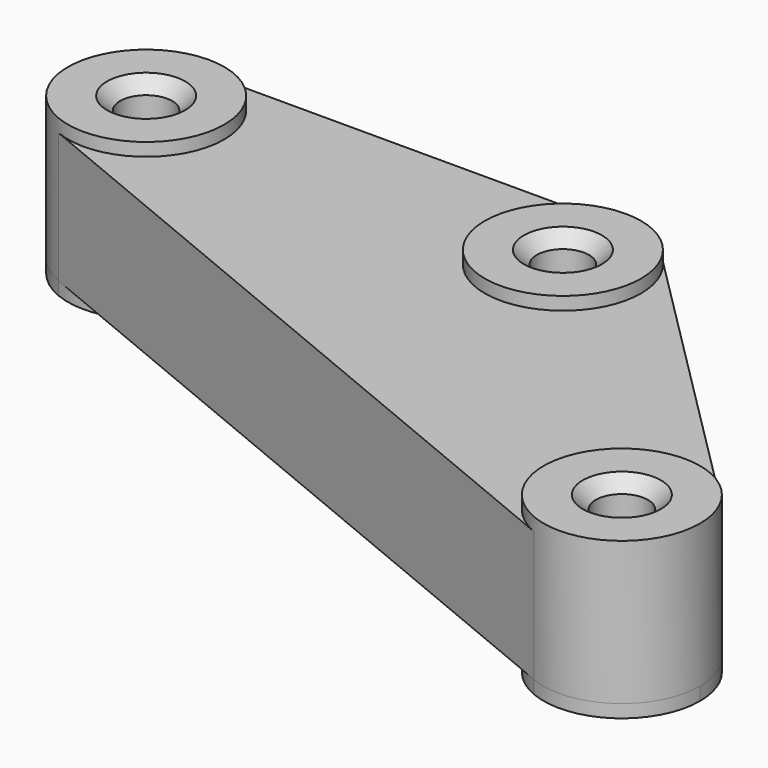
from build123d import *

# Parameters (mm, degrees)
F0_R     = 2
F1_DEPTH = 10
F2_DEPTH = 11
F3_DEPTH = 1


# Not quite as in the source:
# - a fillet or chamfer that OpenCascade refuses, or shapes differently, is made with other operations: its cross-section is extruded or revolved along the edge and cut away or added
# - after a boolean that leaves OpenCascade's solid faulty, fix() repairs it


with BuildPart() as f1:
    # F0 (on Top) → F1 (new body)
    with BuildSketch(Plane.XY):
        with BuildLine():
            Line((26, 0), (6, 0))
            ThreePointArc((6, 0), (3.3334213981, -4.9888176738), (-2.2961005942, -5.5432771951))
            Line((-2.2961005942, -5.5432771951), (52.3313164038, -28.170694193))
            ThreePointArc((52.3313164038, -28.170694193), (48.7427053156, -23.7979589301), (50.3847763109, -18.3847763109))
            Line((50.3847763109, -18.3847763109), (36.2426406871, -4.2426406871))
            ThreePointArc((36.2426406871, -4.2426406871), (29.7038994058, -5.5432771951), (26, 0))
        make_face()
        with BuildLine():
            ThreePointArc((0, 6), (4.2426406871, 4.2426406871), (6, 0))
            Line((6, 0), (26, 0))
            ThreePointArc((26, 0), (27.7573593129, 4.2426406871), (32, 6))
            Line((32, 6), (0, 6))
        make_face()
        with BuildLine():
            ThreePointArc((38, 0), (37.5432771951, -2.2961005942), (36.2426406871, -4.2426406871))
            Line((36.2426406871, -4.2426406871), (50.3847763109, -18.3847763109))
            ThreePointArc((50.3847763109, -18.3847763109), (54.627416998, -16.627416998), (58.8700576851, -18.3847763109))
            Line((58.8700576851, -18.3847763109), (36.2426406871, 4.2426406871))
            ThreePointArc((36.2426406871, 4.2426406871), (37.5432771951, 2.2961005942), (38, 0))
        make_face()
        with BuildLine():
            ThreePointArc((-2.2961005942, -5.5432771951), (3.3334213981, -4.9888176738), (6, 0))
            ThreePointArc((6, 0), (4.2426406871, 4.2426406871), (0, 6))
            ThreePointArc((0, 6), (-5.8847116824, 1.1705419321), (-2.2961005942, -5.5432771951))
        make_face()
        Circle(F0_R, mode=Mode.SUBTRACT)
        with BuildLine():
            Line((30, 0), (26, 0))
            ThreePointArc((26, 0), (29.7038994058, -5.5432771951), (36.2426406871, -4.2426406871))
            Line((36.2426406871, -4.2426406871), (33.4142135624, -1.4142135624))
            ThreePointArc((33.4142135624, -1.4142135624), (31.2346331353, -1.847759065), (30, 0))
        make_face()
        with BuildLine():
            ThreePointArc((32, 6), (27.7573593129, 4.2426406871), (26, 0))
            Line((26, 0), (30, 0))
            ThreePointArc((30, 0), (32, 2), (34, 0))
            ThreePointArc((34, 0), (33.847759065, -0.7653668647), (33.4142135624, -1.4142135624))
            Line((33.4142135624, -1.4142135624), (36.2426406871, -4.2426406871))
            ThreePointArc((36.2426406871, -4.2426406871), (37.5432771951, -2.2961005942), (38, 0))
            ThreePointArc((38, 0), (37.5432771951, 2.2961005942), (36.2426406871, 4.2426406871))
            ThreePointArc((36.2426406871, 4.2426406871), (34.2961005942, 5.5432771951), (32, 6))
        make_face()
        with BuildLine():
            ThreePointArc((50.3847763109, -18.3847763109), (48.7427053156, -23.7979589301), (52.3313164038, -28.170694193))
            ThreePointArc((52.3313164038, -28.170694193), (57.9608383961, -27.6162346718), (60.627416998, -22.627416998))
            ThreePointArc((60.627416998, -22.627416998), (60.170694193, -20.3313164038), (58.8700576851, -18.3847763109))
            ThreePointArc((58.8700576851, -18.3847763109), (54.627416998, -16.627416998), (50.3847763109, -18.3847763109))
        make_face()
        with BuildLine():
            ThreePointArc((56.627416998, -22.627416998), (53.8620501332, -24.475176063), (53.2132034356, -21.2132034356))
            ThreePointArc((53.2132034356, -21.2132034356), (55.3927838627, -20.7796579329), (56.627416998, -22.627416998))
        make_face(mode=Mode.SUBTRACT)
    extrude(amount=F1_DEPTH)

    # F0 (on Top) → F2 (join)
    with BuildSketch(Plane.XY):
        with BuildLine():
            ThreePointArc((-2.2961005942, -5.5432771951), (3.3334213981, -4.9888176738), (6, 0))
            ThreePointArc((6, 0), (4.2426406871, 4.2426406871), (0, 6))
            ThreePointArc((0, 6), (-5.8847116824, 1.1705419321), (-2.2961005942, -5.5432771951))
        make_face()
        Circle(F0_R, mode=Mode.SUBTRACT)
        with BuildLine():
            ThreePointArc((32, 6), (27.7573593129, 4.2426406871), (26, 0))
            Line((26, 0), (30, 0))
            ThreePointArc((30, 0), (32, 2), (34, 0))
            ThreePointArc((34, 0), (33.847759065, -0.7653668647), (33.4142135624, -1.4142135624))
            Line((33.4142135624, -1.4142135624), (36.2426406871, -4.2426406871))
            ThreePointArc((36.2426406871, -4.2426406871), (37.5432771951, -2.2961005942), (38, 0))
            ThreePointArc((38, 0), (37.5432771951, 2.2961005942), (36.2426406871, 4.2426406871))
            ThreePointArc((36.2426406871, 4.2426406871), (34.2961005942, 5.5432771951), (32, 6))
        make_face()
        with BuildLine():
            Line((30, 0), (26, 0))
            ThreePointArc((26, 0), (29.7038994058, -5.5432771951), (36.2426406871, -4.2426406871))
            Line((36.2426406871, -4.2426406871), (33.4142135624, -1.4142135624))
            ThreePointArc((33.4142135624, -1.4142135624), (31.2346331353, -1.847759065), (30, 0))
        make_face()
        with BuildLine():
            ThreePointArc((50.3847763109, -18.3847763109), (48.7427053156, -23.7979589301), (52.3313164038, -28.170694193))
            ThreePointArc((52.3313164038, -28.170694193), (57.9608383961, -27.6162346718), (60.627416998, -22.627416998))
            ThreePointArc((60.627416998, -22.627416998), (60.170694193, -20.3313164038), (58.8700576851, -18.3847763109))
            ThreePointArc((58.8700576851, -18.3847763109), (54.627416998, -16.627416998), (50.3847763109, -18.3847763109))
        make_face()
        with BuildLine():
            ThreePointArc((56.627416998, -22.627416998), (53.8620501332, -24.475176063), (53.2132034356, -21.2132034356))
            ThreePointArc((53.2132034356, -21.2132034356), (55.3927838627, -20.7796579329), (56.627416998, -22.627416998))
        make_face(mode=Mode.SUBTRACT)
    extrude(amount=F2_DEPTH)

    # F0 (on Top) → F3 (join)
    with BuildSketch(Plane.XY):
        with BuildLine():
            ThreePointArc((-2.2961005942, -5.5432771951), (3.3334213981, -4.9888176738), (6, 0))
            ThreePointArc((6, 0), (4.2426406871, 4.2426406871), (0, 6))
            ThreePointArc((0, 6), (-5.8847116824, 1.1705419321), (-2.2961005942, -5.5432771951))
        make_face()
        Circle(F0_R, mode=Mode.SUBTRACT)
        with BuildLine():
            ThreePointArc((32, 6), (27.7573593129, 4.2426406871), (26, 0))
            Line((26, 0), (30, 0))
            ThreePointArc((30, 0), (32, 2), (34, 0))
            ThreePointArc((34, 0), (33.847759065, -0.7653668647), (33.4142135624, -1.4142135624))
            Line((33.4142135624, -1.4142135624), (36.2426406871, -4.2426406871))
            ThreePointArc((36.2426406871, -4.2426406871), (37.5432771951, -2.2961005942), (38, 0))
            ThreePointArc((38, 0), (37.5432771951, 2.2961005942), (36.2426406871, 4.2426406871))
            ThreePointArc((36.2426406871, 4.2426406871), (34.2961005942, 5.5432771951), (32, 6))
        make_face()
        with BuildLine():
            Line((30, 0), (26, 0))
            ThreePointArc((26, 0), (29.7038994058, -5.5432771951), (36.2426406871, -4.2426406871))
            Line((36.2426406871, -4.2426406871), (33.4142135624, -1.4142135624))
            ThreePointArc((33.4142135624, -1.4142135624), (31.2346331353, -1.847759065), (30, 0))
        make_face()
        with BuildLine():
            ThreePointArc((50.3847763109, -18.3847763109), (48.7427053156, -23.7979589301), (52.3313164038, -28.170694193))
            ThreePointArc((52.3313164038, -28.170694193), (57.9608383961, -27.6162346718), (60.627416998, -22.627416998))
            ThreePointArc((60.627416998, -22.627416998), (60.170694193, -20.3313164038), (58.8700576851, -18.3847763109))
            ThreePointArc((58.8700576851, -18.3847763109), (54.627416998, -16.627416998), (50.3847763109, -18.3847763109))
        make_face()
        with BuildLine():
            ThreePointArc((56.627416998, -22.627416998), (53.8620501332, -24.475176063), (53.2132034356, -21.2132034356))
            ThreePointArc((53.2132034356, -21.2132034356), (55.3927838627, -20.7796579329), (56.627416998, -22.627416998))
        make_face(mode=Mode.SUBTRACT)
    extrude(amount=-F3_DEPTH)

    add(f1.part.fix(), mode=Mode.REPLACE)

    # F4: chamfer of 1 on 6 edges, made by hand

    # F4_s1 → F4_t2 (revolve, cut)
    with BuildSketch(Plane.XZ):
        Polygon((3, 11), (2, 10), (2, 11), align=None)
    revolve(axis=Axis((0, 0, 11), (0, 0, 1)), mode=Mode.SUBTRACT)

    # F4_s3 → F4_t4 (revolve, cut)
    with BuildSketch(Plane(origin=(16, 16, 0), x_dir=(0, 0, 1), z_dir=(0.7071067812, 0.7071067812, 0))):
        Polygon((11, 25.627416998), (10, 24.627416998), (11, 24.627416998), align=None)
    revolve(axis=Axis((32, 0, 11), (0, 0, -1)), mode=Mode.SUBTRACT)

    # F4_s5 → F4_t6 (revolve, cut)
    with BuildSketch(Plane(origin=(16, 16, 0), x_dir=(0, 0, 1), z_dir=(-0.7071067812, -0.7071067812, 0))):
        Polygon((11, -51.627416998), (10, -52.627416998), (11, -52.627416998), align=None)
    revolve(axis=Axis((54.627416998, -22.627416998, 11), (0, 0, -1)), mode=Mode.SUBTRACT)

    # F4_s7 → F4_t8 (revolve, cut)
    with BuildSketch(Plane.XZ):
        Polygon((3, -1), (2, 0), (2, -1), align=None)
    revolve(axis=Axis((0, 0, -1), (0, 0, 1)), mode=Mode.SUBTRACT)

    # F4_s9 → F4_t10 (revolve, cut)
    with BuildSketch(Plane(origin=(16, 16, 0), x_dir=(0, 0, 1), z_dir=(0.7071067812, 0.7071067812, 0))):
        Polygon((-1, 25.627416998), (0, 24.627416998), (-1, 24.627416998), align=None)
    revolve(axis=Axis((32, 0, -1), (0, 0, -1)), mode=Mode.SUBTRACT)

    # F4_s11 → F4_t12 (revolve, cut)
    with BuildSketch(Plane(origin=(16, 16, 0), x_dir=(0, 0, 1), z_dir=(-0.7071067812, -0.7071067812, 0))):
        Polygon((-1, -51.627416998), (0, -52.627416998), (-1, -52.627416998), align=None)
    revolve(axis=Axis((54.627416998, -22.627416998, -1), (0, 0, -1)), mode=Mode.SUBTRACT)


solid = f1.part
